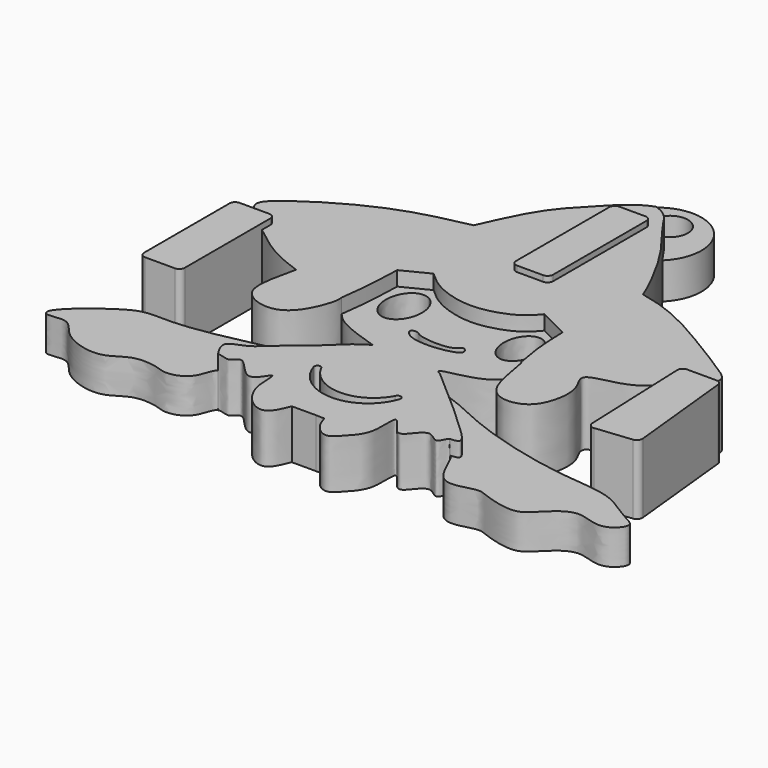
from build123d import *

# Parameters (mm, degrees)
F1_DEPTH = 5.588
F2_DEPTH = 4.318
F3_DEPTH = 3.048
F4_DEPTH = 6.096
F0_R     = 1.5875
F5_DEPTH = 3.175


with BuildPart() as f1:
    # F0 (on Top) → F1 (new body)
    with BuildSketch(Plane.XY):
        with BuildLine():
            add(Edge.make_bspline(
                [(-0.4543650139, 12.2671723366), (0.7606715662, 11.8621597067), (1.1021111017, 11.1123113715), (1.7993424241, 10.1466711624), (1.9588937381, 9.9324109033)],
                knots=[0, 0, 0, 0, 0.2287148556, 0.2901402715, 0.2901402715, 0.2901402715, 0.2901402715], degree=3))
            add(Edge.make_bspline(
                [(-0.4543650139, 12.2671723366), (-1.8212810392, 11.7609063163), (-2.6696978296, 10.8343886176), (-3.5423825029, 9.9324109033)],
                knots=[0, 0, 0, 0, 0.3156742927, 0.3156742927, 0.3156742927, 0.3156742927], degree=3))
            add(Edge.make_bspline(
                [(-3.5423825029, 9.9324109033), (-4.4174746056, 9.0279449505), (-6.3620533051, 7.1259628062), (-7.7468212422, 3.9462225237), (-8.480694145, 2.3120851256)],
                knots=[0.3156742927, 0.3156742927, 0.3156742927, 0.3156742927, 0.6322194195, 1, 1, 1, 1], degree=3))
            add(Edge.make_bspline(
                [(-8.480694145, 2.3120851256), (-9.9427478846, 2.0025585918), (-12.8995772894, 1.3765780742), (-17.0869177602, -0.4039741156), (-20.9657991457, -2.9082685133), (-22.5608107704, -4.4795053921), (-21.6020623487, -5.4020959946), (-21.1244747043, -5.8616721071)],
                knots=[0, 0, 0, 0, 0.2337164826, 0.4726637259, 0.7125914559, 0.8568312954, 1, 1, 1, 1], degree=3))
            Line((-21.1244747043, -5.8616721071), (-19.8688691016, -5.8616721071))
            ThreePointArc((-19.8688691016, -5.8616721071), (-19.5225051481, -6.0051407542), (-19.379036501, -6.3515047077))
            Line((-19.379036501, -6.3515047077), (-19.379036501, -7.2697284631))
            add(Edge.make_bspline(
                [(-19.379036501, -7.2697284631), (-18.4453769662, -8.0037126673), (-16.6548147177, -9.4113397068), (-14.7696376908, -10.0935165723), (-13.8674555346, -10.4199834168)],
                knots=[0, 0, 0, 0, 0.5214337204, 1, 1, 1, 1], degree=3))
            add(Edge.make_bspline(
                [(-13.8674555346, -10.4199834168), (-14.0433557589, -11.1865253996), (-14.3839889341, -12.6709443686), (-14.5389691348, -14.9707773085), (-12.7523382333, -16.0440165388), (-10.8705981999, -15.9682546124), (-9.497511474, -14.4516541705), (-8.7808057491, -12.3378237023), (-8.8367220819, -11.8680504734), (-8.855686523, -11.7087233812)],
                knots=[0, 0, 0, 0, 0.1659663311, 0.3213960561, 0.4658539645, 0.6072212408, 0.7595838646, 0.9184610757, 1, 1, 1, 1], degree=3))
            add(Edge.make_bspline(
                [(-8.855686523, -11.7087233812), (-8.7665463436, -11.0722415209), (-8.5610175103, -9.604717281), (-8.4697703353, -7.3977592962), (-8.4180980921, -6.1479839496)],
                knots=[0, 0, 0, 0, 0.4337113098, 1, 1, 1, 1], degree=3))
            Line((-8.4180980921, -6.1479839496), (-6.1483075842, -5.001142621))
            add(Edge.make_bspline(
                [(-6.1483075842, -5.001142621), (-5.6941276331, -5.4148834114), (-4.718995829, -6.3031916739), (-2.2607149691, -7.1513491175), (-0.0582333694, -7.1239374303), (2.4017473535, -6.2570297819), (3.1786720263, -5.3578494575), (3.5281679593, -4.9533573911)],
                knots=[0, 0, 0, 0, 0.1881579583, 0.4039782225, 0.6081820752, 0.8237425378, 1, 1, 1, 1], degree=3))
            Line((3.5281679593, -4.9533573911), (6.18023891, -6.2674470246))
            add(Edge.make_bspline(
                [(6.7100971937, -11.452040635), (6.5609422348, -10.643335226), (6.2557121704, -8.9884039668), (6.2057740608, -7.1880385752), (6.18023891, -6.2674470246)],
                knots=[0, 0, 0, 0, 0.4886640484, 1, 1, 1, 1], degree=3))
            add(Edge.make_bspline(
                [(16.4709712436, -8.1202534024), (15.8466679007, -8.6963230282), (14.5764628641, -9.8683919406), (10.6912309199, -10.225721996), (12.3009892622, -12.0923969004), (12.1385032422, -14.5630395394), (10.9762657463, -16.663305051), (7.0770353536, -16.7388344061), (7.0362674031, -11.7143300057), (6.7100971937, -11.452040635)],
                knots=[0, 0, 0, 0, 0.0321612874, 0.0654352243, 0.089572823, 0.1202596245, 0.1491615149, 0.1817792541, 0.2230593148, 0.2230593148, 0.2230593148, 0.2230593148], degree=3))
            Line((16.4709712436, -8.1202534024), (16.4081356079, -6.5252292211))
            ThreePointArc((16.4081356079, -6.5252292211), (16.5444732197, -6.1664689948), (16.8975885527, -6.0161147267))
            Line((16.8975885527, -6.0161147267), (18.5001827776, -6.0161147267))
            add(Edge.make_bspline(
                [(6.9601801224, 1.5459908172), (7.6231487815, 1.396895891), (9.0756341649, 1.0702466624), (11.8602139447, -0.191802595), (14.7109803429, -1.9125831369), (17.5875318602, -3.6718920191), (19.3916371402, -4.8766949617), (18.7768420022, -5.6625004511), (18.5001827776, -6.0161147267)],
                knots=[0, 0, 0, 0, 0.1565209713, 0.3429188091, 0.5418579227, 0.7437960592, 0.884707638, 1, 1, 1, 1], degree=3))
            add(Edge.make_bspline(
                [(1.9588937381, 9.9324109033), (2.5594088975, 9.1259836143), (4.3673366115, 6.9047774905), (6.4100828339, 2.9385840306), (6.8264157664, 1.9177075698), (6.9601801224, 1.5459908172)],
                knots=[0.2901402715, 0.2901402715, 0.2901402715, 0.2901402715, 0.5213316827, 0.8332007469, 1, 1, 1, 1], degree=3))
        make_face()
        with BuildLine():
            ThreePointArc((-2.3076904472, 9.4425783027), (-2.1642218001, 9.7889422562), (-1.8178578466, 9.9324109033))
            Line((-1.8178578466, 9.9324109033), (0.4555326304, 9.9324109033))
            ThreePointArc((0.4555326304, 9.9324109033), (0.801896584, 9.7889422562), (0.945365231, 9.4425783027))
            Line((0.945365231, 9.4425783027), (0.945365231, -0.7664946606))
            ThreePointArc((0.945365231, -0.7664946606), (0.801896584, -1.1128586142), (0.4555326304, -1.2563272612))
            Line((0.4555326304, -1.2563272612), (-1.8178578466, -1.2563272612))
            ThreePointArc((-1.8178578466, -1.2563272612), (-2.1642218001, -1.1128586142), (-2.3076904472, -0.7664946606))
            Line((-2.3076904472, -0.7664946606), (-2.3076904472, 9.4425783027))
        make_face(mode=Mode.SUBTRACT)
    extrude(amount=F1_DEPTH)

    # F0 (on Top) → F2 (join)
    with BuildSketch(Plane.XY):
        with BuildLine():
            add(Edge.make_bspline(
                [(6.7100971937, -11.452040635), (6.487132333, -11.2727437179), (5.6301792999, -13.6450174593), (1.7404976831, -13.853984965), (1.6145893605, -14.1338864341)],
                knots=[0.2230593148, 0.2230593148, 0.2230593148, 0.2230593148, 0.2512777194, 0.289358463, 0.289358463, 0.289358463, 0.289358463], degree=3))
            add(Edge.make_bspline(
                [(6.7100971937, -11.452040635), (6.5609422348, -10.643335226), (6.2557121704, -8.9884039668), (6.2057740608, -7.1880385752), (6.18023891, -6.2674470246)],
                knots=[0, 0, 0, 0, 0.4886640484, 1, 1, 1, 1], degree=3))
            Line((6.18023891, -6.2674470246), (3.5281679593, -4.9533573911))
            add(Edge.make_bspline(
                [(-6.1483075842, -5.001142621), (-5.6941276331, -5.4148834114), (-4.718995829, -6.3031916739), (-2.2607149691, -7.1513491175), (-0.0582333694, -7.1239374303), (2.4017473535, -6.2570297819), (3.1786720263, -5.3578494575), (3.5281679593, -4.9533573911)],
                knots=[0, 0, 0, 0, 0.1881579583, 0.4039782225, 0.6081820752, 0.8237425378, 1, 1, 1, 1], degree=3))
            Line((-6.1483075842, -5.001142621), (-8.4180980921, -6.1479839496))
            add(Edge.make_bspline(
                [(-8.855686523, -11.7087233812), (-8.7665463436, -11.0722415209), (-8.5610175103, -9.604717281), (-8.4697703353, -7.3977592962), (-8.4180980921, -6.1479839496)],
                knots=[0, 0, 0, 0, 0.4337113098, 1, 1, 1, 1], degree=3))
            add(Edge.make_bspline(
                [(-8.855686523, -11.7087233812), (-8.6097629931, -11.9702795148), (-8.0494416831, -12.5662187301), (-6.3153080865, -13.3120320728), (-5.0122945477, -13.7308422317), (-4.3383073062, -13.9474729076)],
                knots=[0, 0, 0, 0, 0.2741037786, 0.6245282361, 1, 1, 1, 1], degree=3))
            add(Edge.make_bspline(
                [(-4.3383073062, -13.9474729076), (-4.6904000733, -14.205835988), (-5.0424928404, -14.4641990683), (-5.4950816557, -14.7439409047)],
                knots=[0, 0, 0, 0, 0.0322315917, 0.0322315917, 0.0322315917, 0.0322315917], degree=3))
            add(Edge.make_bspline(
                [(-5.4950816557, -14.7439409047), (-6.0638276002, -15.2996983741), (-7.254460773, -16.4631410067), (-9.6471391793, -18.3031059601), (-10.7838959083, -19.5447998698), (-12.7966204506, -19.9769166995), (-12.0920792278, -21.0840760868), (-11.7340777069, -21.6466616839)],
                knots=[0, 0, 0, 0, 0.2221960168, 0.4651531163, 0.6524823656, 0.8234143899, 1, 1, 1, 1], degree=3))
            add(Edge.make_bspline(
                [(-11.7340777069, -21.6466616839), (-11.4466265879, -21.5349261024), (-10.5509487435, -22.1740133584), (-9.9419811997, -20.5495693256), (-7.9668492333, -24.0381722349), (-6.5989878751, -20.7959149431), (-6.959107072, -23.9439992316), (-5.3818474746, -26.0513885071), (-3.7410962207, -26.4159546848), (-3.2461170524, -25.1879176529), (-2.9729334638, -24.510152638)],
                knots=[0.7209838079, 0.7209838079, 0.7209838079, 0.7209838079, 0.7493662771, 0.774475046, 0.8173763688, 0.8508557834, 0.8873149394, 0.9327285909, 0.9628722861, 1, 1, 1, 1], degree=3))
            Line((-2.9729334638, -24.510152638), (-0.8691768589, -24.510152638))
            Line((-0.8691768589, -24.510152638), (-0.105395251, -24.5283711702))
            add(Edge.make_bspline(
                [(8.4801148623, -21.5357821435), (8.3041185303, -21.590532768), (8.0606100216, -22.8462871035), (6.8610857119, -21.2282384751), (5.8393759917, -22.7339865732), (5.0288986724, -23.3984793778), (3.4282519346, -20.4462681636), (3.9676702316, -24.0888574711), (2.7431105574, -25.4511815948), (1.6106997575, -26.7714057864), (0.2853707924, -25.7359701091), (0.024552307, -24.9299529754), (-0.105395251, -24.5283711702)],
                knots=[0.7691900941, 0.7691900941, 0.7691900941, 0.7691900941, 0.7877144378, 0.808492379, 0.8320772203, 0.849237919, 0.8756845252, 0.9040955727, 0.9323235648, 0.9554125324, 0.9777851921, 1, 1, 1, 1], degree=3))
            add(Edge.make_bspline(
                [(8.5238891177, -21.5327867593), (8.5089105607, -21.530443964), (8.4943134734, -21.5313651036), (8.4801148623, -21.5357821435)],
                knots=[0.7676956314, 0.7676956314, 0.7676956314, 0.7676956314, 0.7691900941, 0.7691900941, 0.7691900941, 0.7691900941], degree=3))
            add(Edge.make_bspline(
                [(1.9248389962, -14.3998998449), (2.6978633353, -15.0628833695), (4.4932474963, -16.6072909024), (7.5484880643, -19.3576282303), (9.7133267355, -21.4330976719), (8.8481846147, -21.5104051993), (8.5238891177, -21.5327867593)],
                knots=[0.0349476797, 0.0349476797, 0.0349476797, 0.0349476797, 0.2958977424, 0.633851857, 0.8637378675, 0.9941387642, 0.9941387642, 0.9941387642, 0.9941387642], degree=3))
            add(Edge.make_bspline(
                [(1.6145893605, -14.1338864341), (1.5798989162, -14.2110052943), (1.7052491534, -14.3002606139), (1.9248389962, -14.3998998449)],
                knots=[0.289358463, 0.289358463, 0.289358463, 0.289358463, 0.2998505249, 0.2998505249, 0.2998505249, 0.2998505249], degree=3))
        make_face()
        with BuildLine():
            ThreePointArc((-5.4623684846, -18.9867243171), (-5.2573856329, -18.6565277163), (-4.9211313017, -18.8514143229))
            ThreePointArc((-4.9211313017, -18.8514143229), (-1.67612616, -20.8526194046), (1.5962657053, -18.8965182751))
            ThreePointArc((1.5962657053, -18.8965182751), (1.9609271061, -18.7045954036), (2.1375028882, -19.076930359))
            ThreePointArc((2.1375028882, -19.076930359), (-1.6952107541, -21.79337461), (-5.4623684846, -18.9867243171))
        make_face(mode=Mode.SUBTRACT)
        with BuildLine():
            add(Edge.make_bspline(
                [(-3.1856338028, -10.5442097411), (-3.0022241374, -10.5772510711), (-2.7249681916, -11.0191367862), (0.3934040122, -11.2198120301), (0.741911756, -10.2187306395), (1.4202382465, -10.9217324463), (0.4144282984, -11.554831255), (-2.8873911864, -11.8407149236), (-3.888535421, -10.6385050255), (-3.3398623454, -10.5164254028), (-3.1856338028, -10.5442097411)],
                knots=[0, 0, 0, 0, 0.0940995446, 0.2930993232, 0.391615713, 0.4766884717, 0.5862879336, 0.803529874, 0.9208720239, 1, 1, 1, 1], degree=3))
        make_face(mode=Mode.SUBTRACT)
        with BuildLine():
            add(Edge.make_bspline(
                [(-6.2438780442, -5.980736576), (-8.9719351639, -5.980736576), (-7.607906604, -9.2062284239), (-6.2438780442, -12.4317202717), (-4.8798494844, -9.2062284239), (-3.5158209245, -5.980736576), (-6.2438780442, -5.980736576)],
                knots=[0, 0, 0, 2.0943951024, 2.0943951024, 4.1887902048, 4.1887902048, 6.2831853072, 6.2831853072, 6.2831853072], degree=2, weights=[1, 0.5, 1, 0.5, 1, 0.5, 1]))
        make_face(mode=Mode.SUBTRACT)
        with BuildLine():
            add(Edge.make_bspline(
                [(3.9104484022, -6.0046287253), (1.4021787407, -6.0046287253), (2.6563135715, -9.0867662802), (3.9104484022, -12.1689038351), (5.1645832329, -9.0867662802), (6.4187180636, -6.0046287253), (3.9104484022, -6.0046287253)],
                knots=[0, 0, 0, 2.0943951024, 2.0943951024, 4.1887902048, 4.1887902048, 6.2831853072, 6.2831853072, 6.2831853072], degree=2, weights=[1, 0.5, 1, 0.5, 1, 0.5, 1]))
        make_face(mode=Mode.SUBTRACT)
    extrude(amount=F2_DEPTH)

    # F0 (on Top) → F3 (join)
    with BuildSketch(Plane.XY):
        with BuildLine():
            add(Edge.make_bspline(
                [(6.7100971937, -11.452040635), (6.487132333, -11.2727437179), (5.6301792999, -13.6450174593), (1.7404976831, -13.853984965), (1.6145893605, -14.1338864341)],
                knots=[0.2230593148, 0.2230593148, 0.2230593148, 0.2230593148, 0.2512777194, 0.289358463, 0.289358463, 0.289358463, 0.289358463], degree=3))
            add(Edge.make_bspline(
                [(6.7100971937, -11.452040635), (6.5609422348, -10.643335226), (6.2557121704, -8.9884039668), (6.2057740608, -7.1880385752), (6.18023891, -6.2674470246)],
                knots=[0, 0, 0, 0, 0.4886640484, 1, 1, 1, 1], degree=3))
            Line((6.18023891, -6.2674470246), (3.5281679593, -4.9533573911))
            add(Edge.make_bspline(
                [(-6.1483075842, -5.001142621), (-5.6941276331, -5.4148834114), (-4.718995829, -6.3031916739), (-2.2607149691, -7.1513491175), (-0.0582333694, -7.1239374303), (2.4017473535, -6.2570297819), (3.1786720263, -5.3578494575), (3.5281679593, -4.9533573911)],
                knots=[0, 0, 0, 0, 0.1881579583, 0.4039782225, 0.6081820752, 0.8237425378, 1, 1, 1, 1], degree=3))
            Line((-6.1483075842, -5.001142621), (-8.4180980921, -6.1479839496))
            add(Edge.make_bspline(
                [(-8.855686523, -11.7087233812), (-8.7665463436, -11.0722415209), (-8.5610175103, -9.604717281), (-8.4697703353, -7.3977592962), (-8.4180980921, -6.1479839496)],
                knots=[0, 0, 0, 0, 0.4337113098, 1, 1, 1, 1], degree=3))
            add(Edge.make_bspline(
                [(-8.855686523, -11.7087233812), (-8.6097629931, -11.9702795148), (-8.0494416831, -12.5662187301), (-6.3153080865, -13.3120320728), (-5.0122945477, -13.7308422317), (-4.3383073062, -13.9474729076)],
                knots=[0, 0, 0, 0, 0.2741037786, 0.6245282361, 1, 1, 1, 1], degree=3))
            add(Edge.make_bspline(
                [(-4.3383073062, -13.9474729076), (-4.6904000733, -14.205835988), (-5.0424928404, -14.4641990683), (-5.4950816557, -14.7439409047)],
                knots=[0, 0, 0, 0, 0.0322315917, 0.0322315917, 0.0322315917, 0.0322315917], degree=3))
            add(Edge.make_bspline(
                [(-5.4950816557, -14.7439409047), (-6.0638276002, -15.2996983741), (-7.254460773, -16.4631410067), (-9.6471391793, -18.3031059601), (-10.7838959083, -19.5447998698), (-12.7966204506, -19.9769166995), (-12.0920792278, -21.0840760868), (-11.7340777069, -21.6466616839)],
                knots=[0, 0, 0, 0, 0.2221960168, 0.4651531163, 0.6524823656, 0.8234143899, 1, 1, 1, 1], degree=3))
            add(Edge.make_bspline(
                [(-11.7340777069, -21.6466616839), (-11.4466265879, -21.5349261024), (-10.5509487435, -22.1740133584), (-9.9419811997, -20.5495693256), (-7.9668492333, -24.0381722349), (-6.5989878751, -20.7959149431), (-6.959107072, -23.9439992316), (-5.3818474746, -26.0513885071), (-3.7410962207, -26.4159546848), (-3.2461170524, -25.1879176529), (-2.9729334638, -24.510152638)],
                knots=[0.7209838079, 0.7209838079, 0.7209838079, 0.7209838079, 0.7493662771, 0.774475046, 0.8173763688, 0.8508557834, 0.8873149394, 0.9327285909, 0.9628722861, 1, 1, 1, 1], degree=3))
            Line((-2.9729334638, -24.510152638), (-0.8691768589, -24.510152638))
            Line((-0.8691768589, -24.510152638), (-0.105395251, -24.5283711702))
            add(Edge.make_bspline(
                [(8.4801148623, -21.5357821435), (8.3041185303, -21.590532768), (8.0606100216, -22.8462871035), (6.8610857119, -21.2282384751), (5.8393759917, -22.7339865732), (5.0288986724, -23.3984793778), (3.4282519346, -20.4462681636), (3.9676702316, -24.0888574711), (2.7431105574, -25.4511815948), (1.6106997575, -26.7714057864), (0.2853707924, -25.7359701091), (0.024552307, -24.9299529754), (-0.105395251, -24.5283711702)],
                knots=[0.7691900941, 0.7691900941, 0.7691900941, 0.7691900941, 0.7877144378, 0.808492379, 0.8320772203, 0.849237919, 0.8756845252, 0.9040955727, 0.9323235648, 0.9554125324, 0.9777851921, 1, 1, 1, 1], degree=3))
            add(Edge.make_bspline(
                [(8.5238891177, -21.5327867593), (8.5089105607, -21.530443964), (8.4943134734, -21.5313651036), (8.4801148623, -21.5357821435)],
                knots=[0.7676956314, 0.7676956314, 0.7676956314, 0.7676956314, 0.7691900941, 0.7691900941, 0.7691900941, 0.7691900941], degree=3))
            add(Edge.make_bspline(
                [(1.9248389962, -14.3998998449), (2.6978633353, -15.0628833695), (4.4932474963, -16.6072909024), (7.5484880643, -19.3576282303), (9.7133267355, -21.4330976719), (8.8481846147, -21.5104051993), (8.5238891177, -21.5327867593)],
                knots=[0.0349476797, 0.0349476797, 0.0349476797, 0.0349476797, 0.2958977424, 0.633851857, 0.8637378675, 0.9941387642, 0.9941387642, 0.9941387642, 0.9941387642], degree=3))
            add(Edge.make_bspline(
                [(1.6145893605, -14.1338864341), (1.5798989162, -14.2110052943), (1.7052491534, -14.3002606139), (1.9248389962, -14.3998998449)],
                knots=[0.289358463, 0.289358463, 0.289358463, 0.289358463, 0.2998505249, 0.2998505249, 0.2998505249, 0.2998505249], degree=3))
        make_face()
        with BuildLine():
            ThreePointArc((-5.4623684846, -18.9867243171), (-5.2573856329, -18.6565277163), (-4.9211313017, -18.8514143229))
            ThreePointArc((-4.9211313017, -18.8514143229), (-1.67612616, -20.8526194046), (1.5962657053, -18.8965182751))
            ThreePointArc((1.5962657053, -18.8965182751), (1.9609271061, -18.7045954036), (2.1375028882, -19.076930359))
            ThreePointArc((2.1375028882, -19.076930359), (-1.6952107541, -21.79337461), (-5.4623684846, -18.9867243171))
        make_face(mode=Mode.SUBTRACT)
        with BuildLine():
            add(Edge.make_bspline(
                [(-3.1856338028, -10.5442097411), (-3.0022241374, -10.5772510711), (-2.7249681916, -11.0191367862), (0.3934040122, -11.2198120301), (0.741911756, -10.2187306395), (1.4202382465, -10.9217324463), (0.4144282984, -11.554831255), (-2.8873911864, -11.8407149236), (-3.888535421, -10.6385050255), (-3.3398623454, -10.5164254028), (-3.1856338028, -10.5442097411)],
                knots=[0, 0, 0, 0, 0.0940995446, 0.2930993232, 0.391615713, 0.4766884717, 0.5862879336, 0.803529874, 0.9208720239, 1, 1, 1, 1], degree=3))
        make_face(mode=Mode.SUBTRACT)
        with BuildLine():
            add(Edge.make_bspline(
                [(-6.2438780442, -5.980736576), (-8.9719351639, -5.980736576), (-7.607906604, -9.2062284239), (-6.2438780442, -12.4317202717), (-4.8798494844, -9.2062284239), (-3.5158209245, -5.980736576), (-6.2438780442, -5.980736576)],
                knots=[0, 0, 0, 2.0943951024, 2.0943951024, 4.1887902048, 4.1887902048, 6.2831853072, 6.2831853072, 6.2831853072], degree=2, weights=[1, 0.5, 1, 0.5, 1, 0.5, 1]))
        make_face(mode=Mode.SUBTRACT)
        with BuildLine():
            add(Edge.make_bspline(
                [(3.9104484022, -6.0046287253), (1.4021787407, -6.0046287253), (2.6563135715, -9.0867662802), (3.9104484022, -12.1689038351), (5.1645832329, -9.0867662802), (6.4187180636, -6.0046287253), (3.9104484022, -6.0046287253)],
                knots=[0, 0, 0, 2.0943951024, 2.0943951024, 4.1887902048, 4.1887902048, 6.2831853072, 6.2831853072, 6.2831853072], degree=2, weights=[1, 0.5, 1, 0.5, 1, 0.5, 1]))
        make_face(mode=Mode.SUBTRACT)
        with BuildLine():
            add(Edge.make_bspline(
                [(1.9248389962, -14.3998998449), (2.2996057499, -14.5699508394), (4.4503981553, -15.2334694581), (7.5319936837, -16.9957166954), (15.7943474574, -19.1533732162), (20.7759266728, -19.1064028641), (23.2030276684, -21.1290540977), (25.1111797525, -21.8014762799), (23.1546741594, -23.87223174), (20.5774791862, -22.1275592957), (18.4205657791, -24.3123057426), (17.1402810676, -25.585368636), (14.0437239886, -24.6203656463), (13.2744251783, -24.1969160394), (11.0063032039, -25.0928106173), (9.6498723027, -24.0356820645), (8.8169466168, -21.5786238678), (8.5238891177, -21.5327867593)],
                knots=[0.2998505249, 0.2998505249, 0.2998505249, 0.2998505249, 0.3177569814, 0.3591689684, 0.4160219562, 0.4596687422, 0.4936586595, 0.5166431045, 0.5427996219, 0.5743117759, 0.6060130704, 0.6319084768, 0.6651966337, 0.6841047194, 0.7122294082, 0.7384562661, 0.7676956314, 0.7676956314, 0.7676956314, 0.7676956314], degree=3))
            add(Edge.make_bspline(
                [(1.9248389962, -14.3998998449), (2.6978633353, -15.0628833695), (4.4932474963, -16.6072909024), (7.5484880643, -19.3576282303), (9.7133267355, -21.4330976719), (8.8481846147, -21.5104051993), (8.5238891177, -21.5327867593)],
                knots=[0.0349476797, 0.0349476797, 0.0349476797, 0.0349476797, 0.2958977424, 0.633851857, 0.8637378675, 0.9941387642, 0.9941387642, 0.9941387642, 0.9941387642], degree=3))
        make_face()
        with BuildLine():
            add(Edge.make_bspline(
                [(-5.4950816557, -14.7439409047), (-6.0638276002, -15.2996983741), (-7.254460773, -16.4631410067), (-9.6471391793, -18.3031059601), (-10.7838959083, -19.5447998698), (-12.7966204506, -19.9769166995), (-12.0920792278, -21.0840760868), (-11.7340777069, -21.6466616839)],
                knots=[0, 0, 0, 0, 0.2221960168, 0.4651531163, 0.6524823656, 0.8234143899, 1, 1, 1, 1], degree=3))
            add(Edge.make_bspline(
                [(-5.4950816557, -14.7439409047), (-6.0804219862, -15.1057354818), (-7.6395296903, -15.928405369), (-10.265297288, -16.4733597638), (-14.0472017528, -17.3375346893), (-18.372736563, -18.1030069175), (-21.0130130082, -17.8290957298), (-22.8834487957, -18.7186707239), (-26.5620817753, -21.5957796187), (-26.2209999035, -22.6676198679), (-24.2721193139, -21.9950520188), (-23.3132420357, -23.8229521411), (-21.2114655823, -24.8460278293), (-19.0946629422, -24.932154358), (-17.5671624447, -23.4934497579), (-15.2867921982, -23.7653916146), (-14.3532537108, -24.2764293082), (-12.2229919685, -23.6069502762), (-12.1051743605, -21.7909112541), (-11.7340777069, -21.6466616839)],
                knots=[0.0322315917, 0.0322315917, 0.0322315917, 0.0322315917, 0.0739172231, 0.1184928423, 0.1725981183, 0.2300697003, 0.2726139629, 0.3131729389, 0.3704709595, 0.390633509, 0.4249598143, 0.4615772893, 0.5028157273, 0.5410114138, 0.5792432341, 0.6185316602, 0.646687685, 0.6843423109, 0.7209838079, 0.7209838079, 0.7209838079, 0.7209838079], degree=3))
        make_face()
    extrude(amount=F3_DEPTH)

    # F0 (on Top) → F4 (join)
    with BuildSketch(Plane.XY):
        with BuildLine():
            Line((-19.8688691016, -5.8616721071), (-21.1244747043, -5.8616721071))
            Line((-21.1244747043, -5.8616721071), (-22.4652236793, -5.8616721071))
            ThreePointArc((-22.4652236793, -5.8616721071), (-22.8115876328, -6.0051407542), (-22.9550562799, -6.3515047077))
            Line((-22.9550562799, -6.3515047077), (-22.9550562799, -15.7167522702))
            ThreePointArc((-22.9550562799, -15.7167522702), (-22.8115876328, -16.0631162238), (-22.4652236793, -16.2065848708))
            Line((-22.4652236793, -16.2065848708), (-19.8688691016, -16.2065848708))
            ThreePointArc((-19.8688691016, -16.2065848708), (-19.5225051481, -16.0631162238), (-19.379036501, -15.7167522702))
            Line((-19.379036501, -15.7167522702), (-19.379036501, -7.2697284631))
            Line((-19.379036501, -7.2697284631), (-19.379036501, -6.3515047077))
            ThreePointArc((-19.379036501, -6.3515047077), (-19.5225051481, -6.0051407542), (-19.8688691016, -5.8616721071))
        make_face()
        with BuildLine():
            Line((19.454543019, -6.0161147267), (18.5001827776, -6.0161147267))
            Line((18.5001827776, -6.0161147267), (16.8975885527, -6.0161147267))
            ThreePointArc((16.8975885527, -6.0161147267), (16.5444732197, -6.1664689948), (16.4081356079, -6.5252292211))
            Line((16.4081356079, -6.5252292211), (16.4709712436, -8.1202534024))
            Line((16.4709712436, -8.1202534024), (16.7934439823, -16.305924002))
            ThreePointArc((16.7934439823, -16.305924002), (16.9620611975, -16.6567777741), (17.3333003038, -16.7738745744))
            Line((17.3333003038, -16.7738745744), (20.4830357087, -16.4480397604))
            ThreePointArc((20.4830357087, -16.4480397604), (20.8127982824, -16.2696921056), (20.9198647983, -15.9104039175))
            Line((20.9198647983, -15.9104039175), (19.9417754853, -6.4555439506))
            ThreePointArc((19.9417754853, -6.4555439506), (19.7826030436, -6.1421993419), (19.454543019, -6.0161147267))
        make_face()
        with BuildLine():
            Line((0.4555326304, 9.9324109033), (-1.8178578466, 9.9324109033))
            ThreePointArc((-1.8178578466, 9.9324109033), (-2.1642218001, 9.7889422562), (-2.3076904472, 9.4425783027))
            Line((-2.3076904472, 9.4425783027), (-2.3076904472, -0.7664946606))
            ThreePointArc((-2.3076904472, -0.7664946606), (-2.1642218001, -1.1128586142), (-1.8178578466, -1.2563272612))
            Line((-1.8178578466, -1.2563272612), (0.4555326304, -1.2563272612))
            ThreePointArc((0.4555326304, -1.2563272612), (0.801896584, -1.1128586142), (0.945365231, -0.7664946606))
            Line((0.945365231, -0.7664946606), (0.945365231, 9.4425783027))
            ThreePointArc((0.945365231, 9.4425783027), (0.801896584, 9.7889422562), (0.4555326304, 9.9324109033))
        make_face()
    extrude(amount=F4_DEPTH)

    # F0 (on Top) → F5 (join)
    with BuildSketch(Plane.XY):
        with BuildLine():
            add(Edge.make_bspline(
                [(-0.4543650139, 12.2671723366), (-1.8212810392, 11.7609063163), (-2.6696978296, 10.8343886176), (-3.5423825029, 9.9324109033)],
                knots=[0, 0, 0, 0, 0.3156742927, 0.3156742927, 0.3156742927, 0.3156742927], degree=3))
            add(Edge.make_bspline(
                [(-0.4543650139, 12.2671723366), (0.7606715662, 11.8621597067), (1.1021111017, 11.1123113715), (1.7993424241, 10.1466711624), (1.9588937381, 9.9324109033)],
                knots=[0, 0, 0, 0, 0.2287148556, 0.2901402715, 0.2901402715, 0.2901402715, 0.2901402715], degree=3))
            ThreePointArc((1.9588937381, 9.9324109033), (-0.7917443824, 16.6764907782), (-3.5423825029, 9.9324109033))
        make_face()
        with Locations((-0.7917443824, 14.1831589863)):
            Circle(F0_R, mode=Mode.SUBTRACT)
    extrude(amount=F5_DEPTH)


solid = f1.part
